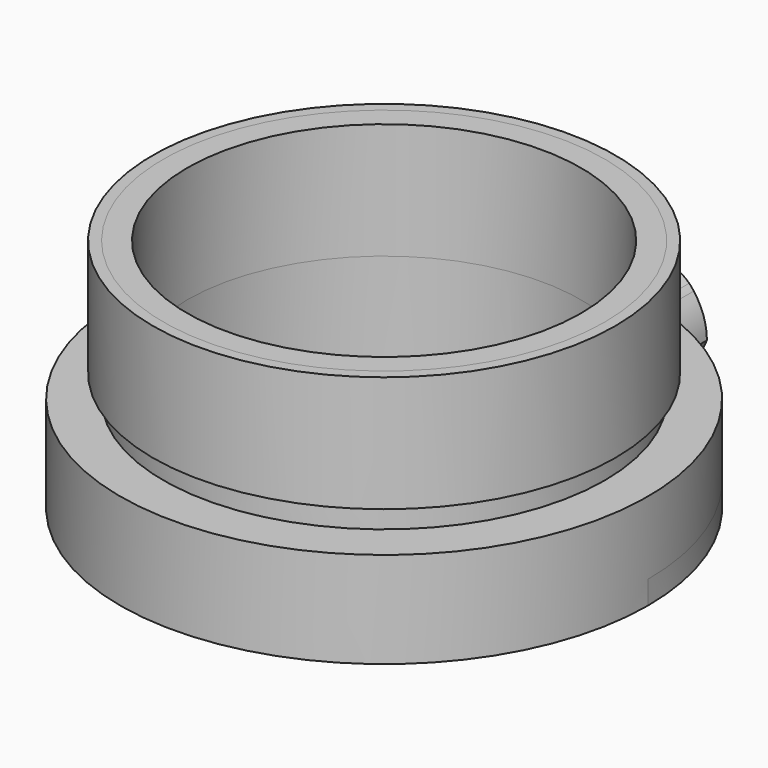
from build123d import *

# Parameters (mm, degrees)
F1_DEPTH  = 2.2
F3_DEPTH  = 8
F4_R      = 5
F5_R      = 18.65
F6_DEPTH  = 5.9
F8_DEPTH  = 8
F9_DEPTH  = 8
F11_DEPTH = 15
F12_DEPTH = 1
F13_R     = 20.9
F13_R_2   = 18.65
F14_DEPTH = 2.2
F15_R     = 21.9
F15_R_2   = 20.9
F16_DEPTH = 11
F17_DEPTH = 11


# Not quite as in the source:
# - a feature names something its author has since deleted; it is built from what else it names


with BuildPart() as f1:
    # F0 (on Top) → F1 (new body)
    with BuildSketch(Plane.XY):
        with BuildLine():
            ThreePointArc((-4.5, 24.5916652547), (-16.0078105936, -19.2028643697), (25, 0))
            ThreePointArc((25, 0), (19.2028643697, 16.0078105936), (4.5, 24.5916652547))
            ThreePointArc((4.5, 24.5916652547), (0, 25), (-4.5, 24.5916652547))
        make_face()
        with BuildLine():
            ThreePointArc((-4.5, 24.5916652547), (0, 25), (4.5, 24.5916652547))
            Line((4.5, 24.5916652547), (4.5, 32.5916652547))
            Line((4.5, 32.5916652547), (-4.5, 32.5916652547))
            Line((-4.5, 32.5916652547), (-4.5, 24.5916652547))
        make_face()
    extrude(amount=F1_DEPTH)

    # F2 (on face) → F3 (cut)
    with BuildSketch(Plane(origin=(0, 32.5916652547, 0), x_dir=(-1, 0, 0), z_dir=(0, 1, 0))):
        Polygon((-3.5, 0), (-4.5, 2.2), (-4.5, 0), align=None)
        Polygon((4.5, 0), (4.5, 2.2), (3.5, 0), align=None)
    extrude(amount=-F3_DEPTH, mode=Mode.SUBTRACT)

    # F4
    f4_edges = [f1.edges().sort_by_distance(p)[0] for p in [
        (-4.5, 24.591665, 1.1),
        (4.5, 24.591665, 1.1),
    ]]
    fillet(f4_edges, radius=F4_R)

    # F5 (on face) → F6 (join)
    with BuildSketch(Plane.XY.offset(2.2)):
        with BuildLine():
            ThreePointArc((-4.5, 24.5686468597), (-4.7640380816, 24.5361130362), (-5.025972006, 24.4895815684))
            ThreePointArc((-5.025972006, 24.4895815684), (0, -25), (5.025972006, 24.4895815684))
            ThreePointArc((5.025972006, 24.4895815684), (4.7640380816, 24.5361130362), (4.5, 24.5686468597))
            Line((4.5, 24.5686468597), (4.5, 32.5916652547))
            Line((4.5, 32.5916652547), (-4.5, 32.5916652547))
            Line((-4.5, 32.5916652547), (-4.5, 24.5686468597))
        make_face()
        Circle(F5_R, mode=Mode.SUBTRACT)
    extrude(amount=F6_DEPTH)

    # F7 (on face) → F8 (cut)
    with BuildSketch(Plane(origin=(0, 32.5916652547, 0), x_dir=(-1, 0, 0), z_dir=(0, 1, 0))):
        with BuildLine():
            Line((-4.5, 8.1), (-4.5, 2.2))
            ThreePointArc((-4.5, 2.2), (-4.1802190183, 4.1520343469), (-3.2543064721, 5.9))
            ThreePointArc((-3.2543064721, 5.9), (-3.0486330946, 6.1637320445), (-2.8216466984, 6.4093604335))
            ThreePointArc((-2.8216466984, 6.4093604335), (-1.5265807136, 7.4478771533), (0, 8.1))
            Line((0, 8.1), (-4.5, 8.1))
        make_face()
        with BuildLine():
            ThreePointArc((3.2543064721, 5.9), (4.1802190183, 4.1520343469), (4.5, 2.2))
            Line((4.5, 2.2), (4.5, 8.1))
            Line((4.5, 8.1), (0, 8.1))
            ThreePointArc((0, 8.1), (1.5265807136, 7.4478771533), (2.8216466984, 6.4093604335))
            ThreePointArc((2.8216466984, 6.4093604335), (3.0486330946, 6.1637320445), (3.2543064721, 5.9))
        make_face()
        with BuildLine():
            ThreePointArc((0, 8.1), (-1.5265807136, 7.4478771533), (-2.8216466984, 6.4093604335))
            ThreePointArc((-2.8216466984, 6.4093604335), (0, 7.5741690978), (2.8216466984, 6.4093604335))
            ThreePointArc((2.8216466984, 6.4093604335), (1.5265807136, 7.4478771533), (0, 8.1))
        make_face()
    extrude(amount=-F8_DEPTH, mode=Mode.SUBTRACT)

    # F7 (on face) → F9 (cut)
    with BuildSketch(Plane(origin=(0, 32.5916652547, 0), x_dir=(-1, 0, 0), z_dir=(0, 1, 0))):
        with BuildLine():
            Line((-4.5, 8.1), (-4.5, 2.2))
            ThreePointArc((-4.5, 2.2), (-4.1802190183, 4.1520343469), (-3.2543064721, 5.9))
            ThreePointArc((-3.2543064721, 5.9), (-3.0486330946, 6.1637320445), (-2.8216466984, 6.4093604335))
            ThreePointArc((-2.8216466984, 6.4093604335), (-1.5265807136, 7.4478771533), (0, 8.1))
            Line((0, 8.1), (-4.5, 8.1))
        make_face()
    extrude(amount=-F9_DEPTH, mode=Mode.SUBTRACT)

    # F10 (on face) → F11 (cut)
    with BuildSketch(Plane(origin=(0, 32.5916652547, 0), x_dir=(-1, 0, 0), z_dir=(0, 1, 0))):
        with BuildLine():
            ThreePointArc((2.5, 2.2), (0, 5.3741690978), (-2.5, 2.2))
            Line((-2.5, 2.2), (2.5, 2.2))
        make_face()
    extrude(amount=-F11_DEPTH, mode=Mode.SUBTRACT)

    # F12 (add): a face of the model
    f12_faces = [f1.faces().sort_by_distance(p)[0] for p in [
        (-3.7957746623, 24.5801560572, 8.1),
    ]]
    extrude(f12_faces, amount=F12_DEPTH)

    # F13 (on face) → F14 (join)
    with BuildSketch(Plane.XY.offset(9.1)):
        Circle(F13_R)
        Circle(F13_R_2, mode=Mode.SUBTRACT)
    extrude(amount=F14_DEPTH)


with BuildPart() as f16:
    # F15 (on face) → F16 (new body)
    with BuildSketch(Plane.XY.offset(11.3)):
        Circle(F15_R)
        Circle(F15_R_2, mode=Mode.SUBTRACT)
    extrude(amount=F16_DEPTH)


with BuildPart() as f17:
    # F17 (new): a face of the model
    f17_faces = [f1.part.faces().sort_by_distance(p)[0] for p in [
        (-20.3088587309, 0, 11.3),
    ]]
    extrude(f17_faces, amount=F17_DEPTH)


solid = Compound([f1.part, f16.part, f17.part])
